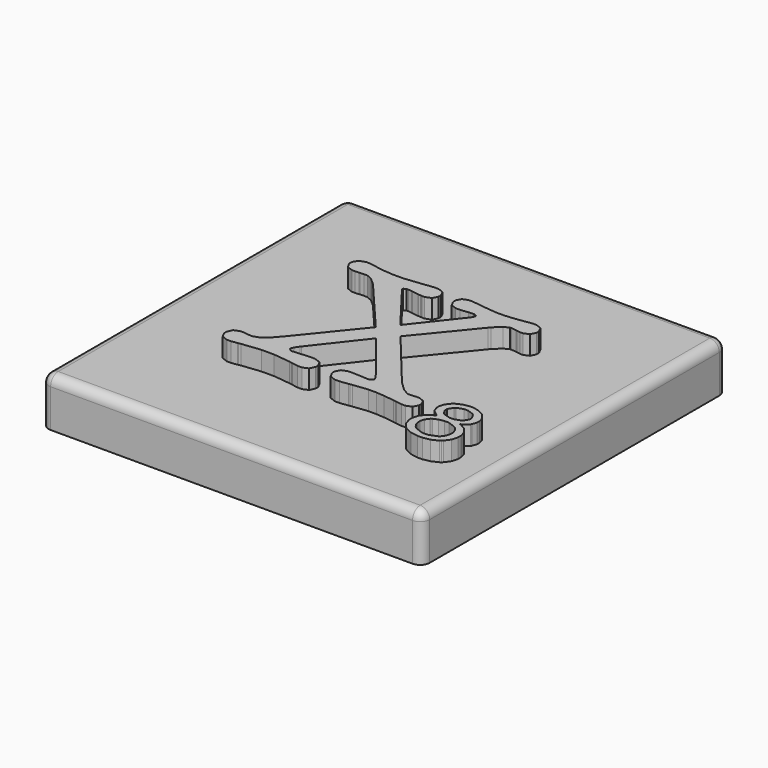
from build123d import *

# Parameters (mm, degrees)
F0_W     = 40
F0_H     = 40
F1_DEPTH = 5
F2_R     = 1
F5_DEPTH = 1
F6_DEPTH = 1
F7_DEPTH = 2


with BuildPart() as f1:
    # F0 (on Top) → F1 (new body)
    with BuildSketch(Plane.XY):
        Rectangle(F0_W, F0_H)
    extrude(amount=-F1_DEPTH)

    # F2
    f2_edges = [f1.edges().sort_by_distance(p)[0] for p in [
        (0, -20, 0),
        (20, 0, 0),
        (0, 20, 0),
        (-20, 0, 0),
        (-20, 20, -2.5),
        (20, 20, -2.5),
        (-20, -20, -2.5),
        (20, -20, -2.5),
    ]]
    fillet(f2_edges, radius=F2_R)

    # F3 (on Top) + F4 (on Top) → F5 (cut)
    with BuildSketch(Plane.XY):
        Polygon((-1.1913108, 0.4106672), (-5.873877, -5.3577998), (-6.0282328, -5.5465726), (-6.678676, -6.2921134), (-7.1651114, -6.7702938), (-7.2367648, -6.8254118), (-7.3098152, -6.8805298), (-8.0208628, -7.1561452), (-8.2813144, -7.1561452), (-8.3901788, -7.1561452), (-8.716772, -7.1230744), (-8.7719154, -7.1175626), (-8.8270334, -7.1106538), (-9.1398344, -7.077583), (-9.2611194, -7.077583), (-9.445752, -7.077583), (-9.9956112, -7.309104), (-10.239502, -7.8299818), (-10.239502, -8.0036416), (-10.239502, -8.1813908), (-9.962515, -8.7174578), (-9.3382846, -8.9558622), (-9.1288108, -8.9558622), (-8.9221056, -8.9558622), (-8.3006184, -8.8662764), (-8.2027776, -8.849741), (-7.960233, -8.8056466), (-6.0006738, -8.5851492), (-5.266182, -8.5851492), (-4.6722538, -8.5851492), (-2.8890722, -8.7835994), (-2.672715, -8.8235536), (-2.5541986, -8.8456008), (-1.8996406, -8.9558622), (-1.6405606, -8.9558622), (-1.4531594, -8.9558622), (-0.8881364, -8.7174578), (-0.6359906, -8.1813908), (-0.6359906, -8.0036416), (-0.6359906, -7.8299818), (-0.9267444, -7.309104), (-1.581277, -7.077583), (-1.7990058, -7.077583), (-1.9478498, -7.077583), (-2.394331, -7.0982586), (-2.4604726, -7.1037704), (-3.2542226, -7.1561452), (-3.86334, -7.2098916), (-3.9156894, -7.2098916), (-4.0094154, -7.2098916), (-4.286377, -6.9907658), (-4.286377, -6.9191124), (-4.286377, -6.8350638), (-4.167886, -6.5870074), (-3.8908736, -6.1722254), (-3.8109906, -6.071616), (0.0530606, -1.124458), (3.9942262, -6.071616), (4.0783002, -6.1763402), (4.371848, -6.6007742), (4.4972224, -6.8391786), (4.4972224, -6.9191124), (4.4972224, -6.985254), (4.1789096, -7.1837042), (4.07416, -7.1837042), (3.8895274, -7.1837042), (3.068193, -7.1299578), (2.9923994, -7.124446), (2.3943564, -7.1037704), (2.1697442, -7.1037704), (1.9657568, -7.1037704), (1.3553186, -7.3283826), (1.083818, -7.834122), (1.083818, -8.0036416), (1.083818, -8.1813908), (1.3676884, -8.7174578), (2.0084796, -8.9558622), (2.2220936, -8.9558622), (2.505964, -8.9558622), (3.3603692, -8.8456008), (3.4926524, -8.8235536), (3.7034724, -8.7877396), (5.2372514, -8.6113366), (5.8201306, -8.6113366), (6.0930028, -8.6113366), (6.9115686, -8.6705948), (8.0291178, -8.8097868), (8.2813144, -8.849741), (8.3915758, -8.8662764), (8.975852, -8.9558622), (9.207373, -8.9558622), (9.4003114, -8.9558622), (9.9804474, -8.7243412), (10.2395274, -8.203438), (10.2395274, -8.0298036), (10.2395274, -7.8658212), (9.9942396, -7.373874), (9.4430342, -7.1561452), (9.2597224, -7.1561452), (9.16051, -7.1561452), (8.8628474, -7.1781924), (8.83666, -7.1837042), (8.6781894, -7.1837042), (8.6561422, -7.187819), (8.5376258, -7.2098916), (8.4921344, -7.2098916), (8.256524, -7.2098916), (7.5537314, -6.8130166), (6.5918334, -5.886958), (6.3754762, -5.6223916), (1.4021562, 0.4106672), (6.058535, 6.0992258), (6.2128908, 6.2893702), (6.9115686, 6.952234), (7.4420984, 7.236079), (7.619873, 7.236079), (8.1131918, 7.1809864), (8.1752186, 7.1699374), (8.2358484, 7.1589392), (8.5913722, 7.1037958), (8.7305642, 7.1037958), (8.9138506, 7.1037958), (9.4650814, 7.3353168), (9.7103692, 7.85622), (9.7103692, 8.029829), (9.7103692, 8.2034634), (9.4374716, 8.724392), (8.8270334, 8.9558622), (8.624443, 8.9558622), (8.439785, 8.9558622), (7.8885796, 8.869045), (7.7783436, 8.8511634), (7.5302872, 8.8112092), (6.4609218, 8.6720172), (5.7223152, 8.612759), (5.4770274, 8.612759), (4.8913542, 8.612759), (3.1385002, 8.789162), (2.9358844, 8.823579), (2.8339542, 8.8415114), (2.182114, 8.9297002), (1.9313144, 8.9297002), (1.7466564, 8.9297002), (1.1954256, 8.7119714), (0.9515094, 8.2213958), (0.9515094, 8.0574134), (0.9515094, 7.883779), (1.2161012, 7.3628758), (1.8114264, 7.1313802), (2.0098512, 7.1313802), (2.2813518, 7.1313802), (3.0998922, 7.219569), (3.2280606, 7.236079), (3.2583628, 7.2416162), (3.5256978, 7.2636634), (3.6249356, 7.2636634), (3.7103812, 7.2636634), (3.9680642, 7.1051674), (3.9680642, 7.0514464), (3.9680642, 6.9439536), (3.7916612, 6.618732), (3.7572442, 6.5746122), (0.1315974, 1.9720052), (-3.5463988, 6.7868546), (-3.5725608, 6.822694), (-3.7048694, 7.025259), (-3.7048694, 7.1037958), (-3.7048694, 7.1506842), (-3.466465, 7.2898508), (-3.3865058, 7.2898508), (-3.2693864, 7.2898508), (-2.9138626, 7.2457564), (-2.8449778, 7.236079), (-2.7774392, 7.227824), (-2.1490432, 7.1410068), (-2.091182, 7.1313802), (-1.8527776, 7.1313802), (-1.8266156, 7.1272146), (-1.675003, 7.1037958), (-1.6143732, 7.1037958), (-1.415923, 7.1037958), (-0.8206232, 7.3353168), (-0.5560314, 7.85622), (-0.5560314, 8.029829), (-0.5560314, 8.1993486), (-0.8206232, 8.705088), (-1.415923, 8.9297002), (-1.6143732, 8.9297002), (-1.8238216, 8.9297002), (-2.4522176, 8.8649302), (-2.5404064, 8.8511634), (-2.8270454, 8.807069), (-4.8830738, 8.586597), (-5.663057, 8.586597), (-6.003417, 8.586597), (-7.0218046, 8.6747858), (-7.1444358, 8.6912958), (-7.4007472, 8.7353902), (-8.3281774, 8.8897206), (-8.69061, 8.9558622), (-8.810498, 8.9558622), (-9.0240866, 8.9558622), (-9.6648778, 8.732647), (-9.9487482, 8.2268822), (-9.9487482, 8.0574134), (-9.9487482, 7.8796642), (-9.6786446, 7.3435718), (-9.068181, 7.1037958), (-8.8642444, 7.1037958), (-8.7319358, 7.1037958), (-8.3336892, 7.1272146), (-8.2689192, 7.1313802), (-8.2055208, 7.135495), (-7.822438, 7.1575422), (-7.673594, 7.1575422), (-7.4793094, 7.1575422), (-6.8936362, 6.8929758), (-6.1825632, 6.2756034), (-6.0323476, 6.0992258), align=None)
    with BuildSketch(Plane.XY):
        Polygon((11.9091701338, -9.0316077608), (11.8678189338, -9.0633069608), (11.7562113338, -9.1487525608), (11.3675913338, -9.6696303608), (11.2022373338, -10.2649555608), (11.2022373338, -10.4633803608), (11.2022373338, -10.6728541608), (11.3772433338, -11.3039933608), (11.7879105338, -11.8648507608), (11.9064015338, -11.9585513608), (12.0235463338, -12.0522773608), (12.7277105338, -12.3802421608), (13.5187173338, -12.5208057608), (13.7833091338, -12.5208057608), (14.0368519338, -12.5208057608), (14.7989027338, -12.3774989608), (15.4851599338, -12.0439969608), (15.6023301338, -11.9489247608), (15.7180779338, -11.8538271608), (16.1232079338, -11.2915981608), (16.2968423338, -10.6700855608), (16.2968423338, -10.4633803608), (16.2968423338, -10.2635839608), (16.1301167338, -9.6655155608), (15.7414967338, -9.1473555608), (15.6312607338, -9.0633069608), (15.5871409338, -9.0316077608), (15.0400757338, -8.7449687608), (14.9739087338, -8.7201783608), (15.0593543338, -8.6705721608), (15.6505393338, -8.1978781608), (15.6836101338, -8.1537837608), (15.7153093338, -8.1083177608), (15.8779201338, -7.6287911608), (15.8779201338, -7.4537597608), (15.8779201338, -7.2870087608), (15.7235643338, -6.7881527608), (15.3652973338, -6.3209959608), (15.2632909338, -6.2397159608), (15.1599637338, -6.1570389608), (14.5784307338, -5.8703999608), (13.9596867338, -5.7491149608), (13.7543531338, -5.7491149608), (13.5476479338, -5.7491149608), (12.9289039338, -5.8703999608), (12.3459993338, -6.1570389608), (12.2440183338, -6.2397159608), (12.1406657338, -6.3209959608), (11.7837703338, -6.7881527608), (11.6308115338, -7.2870087608), (11.6308115338, -7.4537597608), (11.6308115338, -7.6163705608), (11.7892821338, -8.1083177608), (11.8209813338, -8.1537837608), (11.8526551338, -8.1978781608), (12.4466087338, -8.6705721608), (12.5347975338, -8.7201783608), (12.4645157338, -8.7449687608), align=None)
        Polygon((13.6096747338, -9.0825855608), (13.7929357338, -9.0825855608), (14.0754345338, -9.0825855608), (14.9243279338, -9.3954119608), (15.0014677338, -9.4588103608), (15.0772867338, -9.5208117608), (15.3446217338, -9.8956395608), (15.4589979338, -10.3131901608), (15.4589979338, -10.4537537608), (15.4589979338, -10.5929203608), (15.3404815338, -11.0146111608), (15.0662377338, -11.3935791608), (14.9877009338, -11.4583237608), (14.9091387338, -11.5217221608), (14.0616677338, -11.8441751608), (13.7543531338, -11.8441751608), (13.4649709338, -11.8441751608), (12.5995675338, -11.5217221608), (12.5210053338, -11.4583237608), (12.4424685338, -11.3935791608), (12.1668531338, -11.0146111608), (12.0497337338, -10.5929203608), (12.0497337338, -10.4537537608), (12.0497337338, -10.3104215608), (12.1641099338, -9.8832443608), (12.4341881338, -9.5097881608), (12.5113787338, -9.4491583608), (12.5871723338, -9.3871569608), (13.0612125338, -9.1735429608), align=None, mode=Mode.SUBTRACT)
        Polygon((13.5187173338, -6.4243485608), (13.7543531338, -6.4243485608), (13.9707103338, -6.4243485608), (14.6211535338, -6.6627783608), (14.6831549338, -6.7109875608), (14.7438101338, -6.7578505608), (15.0497277338, -7.2608213608), (15.0497277338, -7.4441077608), (15.0497277338, -7.5984381608), (14.7520651338, -8.0628263608), (14.6927815338, -8.1055491608), (14.6321771338, -8.1469003608), (13.9886173338, -8.3591427608), (13.7543531338, -8.3591427608), (13.5324841338, -8.3591427608), (12.8710427338, -8.1469003608), (12.8117845338, -8.1055491608), (12.7511547338, -8.0628263608), (12.4493519338, -7.6163705608), (12.4493519338, -7.4537597608), (12.4493519338, -7.2801253608), (12.7538979338, -6.7633369608), (12.8159247338, -6.7151277608), (12.8765545338, -6.6668931608), align=None, mode=Mode.SUBTRACT)
    extrude(amount=-F5_DEPTH, mode=Mode.SUBTRACT)


with BuildPart() as f6:
    # F3 (on Top) → F6 (new body)
    with BuildSketch(Plane.XY):
        Polygon((-1.1913108, 0.4106672), (-5.873877, -5.3577998), (-6.0282328, -5.5465726), (-6.678676, -6.2921134), (-7.1651114, -6.7702938), (-7.2367648, -6.8254118), (-7.3098152, -6.8805298), (-8.0208628, -7.1561452), (-8.2813144, -7.1561452), (-8.3901788, -7.1561452), (-8.716772, -7.1230744), (-8.7719154, -7.1175626), (-8.8270334, -7.1106538), (-9.1398344, -7.077583), (-9.2611194, -7.077583), (-9.445752, -7.077583), (-9.9956112, -7.309104), (-10.239502, -7.8299818), (-10.239502, -8.0036416), (-10.239502, -8.1813908), (-9.962515, -8.7174578), (-9.3382846, -8.9558622), (-9.1288108, -8.9558622), (-8.9221056, -8.9558622), (-8.3006184, -8.8662764), (-8.2027776, -8.849741), (-7.960233, -8.8056466), (-6.0006738, -8.5851492), (-5.266182, -8.5851492), (-4.6722538, -8.5851492), (-2.8890722, -8.7835994), (-2.672715, -8.8235536), (-2.5541986, -8.8456008), (-1.8996406, -8.9558622), (-1.6405606, -8.9558622), (-1.4531594, -8.9558622), (-0.8881364, -8.7174578), (-0.6359906, -8.1813908), (-0.6359906, -8.0036416), (-0.6359906, -7.8299818), (-0.9267444, -7.309104), (-1.581277, -7.077583), (-1.7990058, -7.077583), (-1.9478498, -7.077583), (-2.394331, -7.0982586), (-2.4604726, -7.1037704), (-3.2542226, -7.1561452), (-3.86334, -7.2098916), (-3.9156894, -7.2098916), (-4.0094154, -7.2098916), (-4.286377, -6.9907658), (-4.286377, -6.9191124), (-4.286377, -6.8350638), (-4.167886, -6.5870074), (-3.8908736, -6.1722254), (-3.8109906, -6.071616), (0.0530606, -1.124458), (3.9942262, -6.071616), (4.0783002, -6.1763402), (4.371848, -6.6007742), (4.4972224, -6.8391786), (4.4972224, -6.9191124), (4.4972224, -6.985254), (4.1789096, -7.1837042), (4.07416, -7.1837042), (3.8895274, -7.1837042), (3.068193, -7.1299578), (2.9923994, -7.124446), (2.3943564, -7.1037704), (2.1697442, -7.1037704), (1.9657568, -7.1037704), (1.3553186, -7.3283826), (1.083818, -7.834122), (1.083818, -8.0036416), (1.083818, -8.1813908), (1.3676884, -8.7174578), (2.0084796, -8.9558622), (2.2220936, -8.9558622), (2.505964, -8.9558622), (3.3603692, -8.8456008), (3.4926524, -8.8235536), (3.7034724, -8.7877396), (5.2372514, -8.6113366), (5.8201306, -8.6113366), (6.0930028, -8.6113366), (6.9115686, -8.6705948), (8.0291178, -8.8097868), (8.2813144, -8.849741), (8.3915758, -8.8662764), (8.975852, -8.9558622), (9.207373, -8.9558622), (9.4003114, -8.9558622), (9.9804474, -8.7243412), (10.2395274, -8.203438), (10.2395274, -8.0298036), (10.2395274, -7.8658212), (9.9942396, -7.373874), (9.4430342, -7.1561452), (9.2597224, -7.1561452), (9.16051, -7.1561452), (8.8628474, -7.1781924), (8.83666, -7.1837042), (8.6781894, -7.1837042), (8.6561422, -7.187819), (8.5376258, -7.2098916), (8.4921344, -7.2098916), (8.256524, -7.2098916), (7.5537314, -6.8130166), (6.5918334, -5.886958), (6.3754762, -5.6223916), (1.4021562, 0.4106672), (6.058535, 6.0992258), (6.2128908, 6.2893702), (6.9115686, 6.952234), (7.4420984, 7.236079), (7.619873, 7.236079), (8.1131918, 7.1809864), (8.1752186, 7.1699374), (8.2358484, 7.1589392), (8.5913722, 7.1037958), (8.7305642, 7.1037958), (8.9138506, 7.1037958), (9.4650814, 7.3353168), (9.7103692, 7.85622), (9.7103692, 8.029829), (9.7103692, 8.2034634), (9.4374716, 8.724392), (8.8270334, 8.9558622), (8.624443, 8.9558622), (8.439785, 8.9558622), (7.8885796, 8.869045), (7.7783436, 8.8511634), (7.5302872, 8.8112092), (6.4609218, 8.6720172), (5.7223152, 8.612759), (5.4770274, 8.612759), (4.8913542, 8.612759), (3.1385002, 8.789162), (2.9358844, 8.823579), (2.8339542, 8.8415114), (2.182114, 8.9297002), (1.9313144, 8.9297002), (1.7466564, 8.9297002), (1.1954256, 8.7119714), (0.9515094, 8.2213958), (0.9515094, 8.0574134), (0.9515094, 7.883779), (1.2161012, 7.3628758), (1.8114264, 7.1313802), (2.0098512, 7.1313802), (2.2813518, 7.1313802), (3.0998922, 7.219569), (3.2280606, 7.236079), (3.2583628, 7.2416162), (3.5256978, 7.2636634), (3.6249356, 7.2636634), (3.7103812, 7.2636634), (3.9680642, 7.1051674), (3.9680642, 7.0514464), (3.9680642, 6.9439536), (3.7916612, 6.618732), (3.7572442, 6.5746122), (0.1315974, 1.9720052), (-3.5463988, 6.7868546), (-3.5725608, 6.822694), (-3.7048694, 7.025259), (-3.7048694, 7.1037958), (-3.7048694, 7.1506842), (-3.466465, 7.2898508), (-3.3865058, 7.2898508), (-3.2693864, 7.2898508), (-2.9138626, 7.2457564), (-2.8449778, 7.236079), (-2.7774392, 7.227824), (-2.1490432, 7.1410068), (-2.091182, 7.1313802), (-1.8527776, 7.1313802), (-1.8266156, 7.1272146), (-1.675003, 7.1037958), (-1.6143732, 7.1037958), (-1.415923, 7.1037958), (-0.8206232, 7.3353168), (-0.5560314, 7.85622), (-0.5560314, 8.029829), (-0.5560314, 8.1993486), (-0.8206232, 8.705088), (-1.415923, 8.9297002), (-1.6143732, 8.9297002), (-1.8238216, 8.9297002), (-2.4522176, 8.8649302), (-2.5404064, 8.8511634), (-2.8270454, 8.807069), (-4.8830738, 8.586597), (-5.663057, 8.586597), (-6.003417, 8.586597), (-7.0218046, 8.6747858), (-7.1444358, 8.6912958), (-7.4007472, 8.7353902), (-8.3281774, 8.8897206), (-8.69061, 8.9558622), (-8.810498, 8.9558622), (-9.0240866, 8.9558622), (-9.6648778, 8.732647), (-9.9487482, 8.2268822), (-9.9487482, 8.0574134), (-9.9487482, 7.8796642), (-9.6786446, 7.3435718), (-9.068181, 7.1037958), (-8.8642444, 7.1037958), (-8.7319358, 7.1037958), (-8.3336892, 7.1272146), (-8.2689192, 7.1313802), (-8.2055208, 7.135495), (-7.822438, 7.1575422), (-7.673594, 7.1575422), (-7.4793094, 7.1575422), (-6.8936362, 6.8929758), (-6.1825632, 6.2756034), (-6.0323476, 6.0992258), align=None)
    extrude(amount=-F6_DEPTH)

    # F3 (on Top) → F7 (join)
    with BuildSketch(Plane.XY):
        Polygon((-1.1913108, 0.4106672), (-5.873877, -5.3577998), (-6.0282328, -5.5465726), (-6.678676, -6.2921134), (-7.1651114, -6.7702938), (-7.2367648, -6.8254118), (-7.3098152, -6.8805298), (-8.0208628, -7.1561452), (-8.2813144, -7.1561452), (-8.3901788, -7.1561452), (-8.716772, -7.1230744), (-8.7719154, -7.1175626), (-8.8270334, -7.1106538), (-9.1398344, -7.077583), (-9.2611194, -7.077583), (-9.445752, -7.077583), (-9.9956112, -7.309104), (-10.239502, -7.8299818), (-10.239502, -8.0036416), (-10.239502, -8.1813908), (-9.962515, -8.7174578), (-9.3382846, -8.9558622), (-9.1288108, -8.9558622), (-8.9221056, -8.9558622), (-8.3006184, -8.8662764), (-8.2027776, -8.849741), (-7.960233, -8.8056466), (-6.0006738, -8.5851492), (-5.266182, -8.5851492), (-4.6722538, -8.5851492), (-2.8890722, -8.7835994), (-2.672715, -8.8235536), (-2.5541986, -8.8456008), (-1.8996406, -8.9558622), (-1.6405606, -8.9558622), (-1.4531594, -8.9558622), (-0.8881364, -8.7174578), (-0.6359906, -8.1813908), (-0.6359906, -8.0036416), (-0.6359906, -7.8299818), (-0.9267444, -7.309104), (-1.581277, -7.077583), (-1.7990058, -7.077583), (-1.9478498, -7.077583), (-2.394331, -7.0982586), (-2.4604726, -7.1037704), (-3.2542226, -7.1561452), (-3.86334, -7.2098916), (-3.9156894, -7.2098916), (-4.0094154, -7.2098916), (-4.286377, -6.9907658), (-4.286377, -6.9191124), (-4.286377, -6.8350638), (-4.167886, -6.5870074), (-3.8908736, -6.1722254), (-3.8109906, -6.071616), (0.0530606, -1.124458), (3.9942262, -6.071616), (4.0783002, -6.1763402), (4.371848, -6.6007742), (4.4972224, -6.8391786), (4.4972224, -6.9191124), (4.4972224, -6.985254), (4.1789096, -7.1837042), (4.07416, -7.1837042), (3.8895274, -7.1837042), (3.068193, -7.1299578), (2.9923994, -7.124446), (2.3943564, -7.1037704), (2.1697442, -7.1037704), (1.9657568, -7.1037704), (1.3553186, -7.3283826), (1.083818, -7.834122), (1.083818, -8.0036416), (1.083818, -8.1813908), (1.3676884, -8.7174578), (2.0084796, -8.9558622), (2.2220936, -8.9558622), (2.505964, -8.9558622), (3.3603692, -8.8456008), (3.4926524, -8.8235536), (3.7034724, -8.7877396), (5.2372514, -8.6113366), (5.8201306, -8.6113366), (6.0930028, -8.6113366), (6.9115686, -8.6705948), (8.0291178, -8.8097868), (8.2813144, -8.849741), (8.3915758, -8.8662764), (8.975852, -8.9558622), (9.207373, -8.9558622), (9.4003114, -8.9558622), (9.9804474, -8.7243412), (10.2395274, -8.203438), (10.2395274, -8.0298036), (10.2395274, -7.8658212), (9.9942396, -7.373874), (9.4430342, -7.1561452), (9.2597224, -7.1561452), (9.16051, -7.1561452), (8.8628474, -7.1781924), (8.83666, -7.1837042), (8.6781894, -7.1837042), (8.6561422, -7.187819), (8.5376258, -7.2098916), (8.4921344, -7.2098916), (8.256524, -7.2098916), (7.5537314, -6.8130166), (6.5918334, -5.886958), (6.3754762, -5.6223916), (1.4021562, 0.4106672), (6.058535, 6.0992258), (6.2128908, 6.2893702), (6.9115686, 6.952234), (7.4420984, 7.236079), (7.619873, 7.236079), (8.1131918, 7.1809864), (8.1752186, 7.1699374), (8.2358484, 7.1589392), (8.5913722, 7.1037958), (8.7305642, 7.1037958), (8.9138506, 7.1037958), (9.4650814, 7.3353168), (9.7103692, 7.85622), (9.7103692, 8.029829), (9.7103692, 8.2034634), (9.4374716, 8.724392), (8.8270334, 8.9558622), (8.624443, 8.9558622), (8.439785, 8.9558622), (7.8885796, 8.869045), (7.7783436, 8.8511634), (7.5302872, 8.8112092), (6.4609218, 8.6720172), (5.7223152, 8.612759), (5.4770274, 8.612759), (4.8913542, 8.612759), (3.1385002, 8.789162), (2.9358844, 8.823579), (2.8339542, 8.8415114), (2.182114, 8.9297002), (1.9313144, 8.9297002), (1.7466564, 8.9297002), (1.1954256, 8.7119714), (0.9515094, 8.2213958), (0.9515094, 8.0574134), (0.9515094, 7.883779), (1.2161012, 7.3628758), (1.8114264, 7.1313802), (2.0098512, 7.1313802), (2.2813518, 7.1313802), (3.0998922, 7.219569), (3.2280606, 7.236079), (3.2583628, 7.2416162), (3.5256978, 7.2636634), (3.6249356, 7.2636634), (3.7103812, 7.2636634), (3.9680642, 7.1051674), (3.9680642, 7.0514464), (3.9680642, 6.9439536), (3.7916612, 6.618732), (3.7572442, 6.5746122), (0.1315974, 1.9720052), (-3.5463988, 6.7868546), (-3.5725608, 6.822694), (-3.7048694, 7.025259), (-3.7048694, 7.1037958), (-3.7048694, 7.1506842), (-3.466465, 7.2898508), (-3.3865058, 7.2898508), (-3.2693864, 7.2898508), (-2.9138626, 7.2457564), (-2.8449778, 7.236079), (-2.7774392, 7.227824), (-2.1490432, 7.1410068), (-2.091182, 7.1313802), (-1.8527776, 7.1313802), (-1.8266156, 7.1272146), (-1.675003, 7.1037958), (-1.6143732, 7.1037958), (-1.415923, 7.1037958), (-0.8206232, 7.3353168), (-0.5560314, 7.85622), (-0.5560314, 8.029829), (-0.5560314, 8.1993486), (-0.8206232, 8.705088), (-1.415923, 8.9297002), (-1.6143732, 8.9297002), (-1.8238216, 8.9297002), (-2.4522176, 8.8649302), (-2.5404064, 8.8511634), (-2.8270454, 8.807069), (-4.8830738, 8.586597), (-5.663057, 8.586597), (-6.003417, 8.586597), (-7.0218046, 8.6747858), (-7.1444358, 8.6912958), (-7.4007472, 8.7353902), (-8.3281774, 8.8897206), (-8.69061, 8.9558622), (-8.810498, 8.9558622), (-9.0240866, 8.9558622), (-9.6648778, 8.732647), (-9.9487482, 8.2268822), (-9.9487482, 8.0574134), (-9.9487482, 7.8796642), (-9.6786446, 7.3435718), (-9.068181, 7.1037958), (-8.8642444, 7.1037958), (-8.7319358, 7.1037958), (-8.3336892, 7.1272146), (-8.2689192, 7.1313802), (-8.2055208, 7.135495), (-7.822438, 7.1575422), (-7.673594, 7.1575422), (-7.4793094, 7.1575422), (-6.8936362, 6.8929758), (-6.1825632, 6.2756034), (-6.0323476, 6.0992258), align=None)
    extrude(amount=F7_DEPTH)


with BuildPart() as f6b:
    # F4 (on Top) → F6, piece 2 (new body)
    with BuildSketch(Plane.XY):
        Polygon((11.9091701338, -9.0316077608), (11.8678189338, -9.0633069608), (11.7562113338, -9.1487525608), (11.3675913338, -9.6696303608), (11.2022373338, -10.2649555608), (11.2022373338, -10.4633803608), (11.2022373338, -10.6728541608), (11.3772433338, -11.3039933608), (11.7879105338, -11.8648507608), (11.9064015338, -11.9585513608), (12.0235463338, -12.0522773608), (12.7277105338, -12.3802421608), (13.5187173338, -12.5208057608), (13.7833091338, -12.5208057608), (14.0368519338, -12.5208057608), (14.7989027338, -12.3774989608), (15.4851599338, -12.0439969608), (15.6023301338, -11.9489247608), (15.7180779338, -11.8538271608), (16.1232079338, -11.2915981608), (16.2968423338, -10.6700855608), (16.2968423338, -10.4633803608), (16.2968423338, -10.2635839608), (16.1301167338, -9.6655155608), (15.7414967338, -9.1473555608), (15.6312607338, -9.0633069608), (15.5871409338, -9.0316077608), (15.0400757338, -8.7449687608), (14.9739087338, -8.7201783608), (15.0593543338, -8.6705721608), (15.6505393338, -8.1978781608), (15.6836101338, -8.1537837608), (15.7153093338, -8.1083177608), (15.8779201338, -7.6287911608), (15.8779201338, -7.4537597608), (15.8779201338, -7.2870087608), (15.7235643338, -6.7881527608), (15.3652973338, -6.3209959608), (15.2632909338, -6.2397159608), (15.1599637338, -6.1570389608), (14.5784307338, -5.8703999608), (13.9596867338, -5.7491149608), (13.7543531338, -5.7491149608), (13.5476479338, -5.7491149608), (12.9289039338, -5.8703999608), (12.3459993338, -6.1570389608), (12.2440183338, -6.2397159608), (12.1406657338, -6.3209959608), (11.7837703338, -6.7881527608), (11.6308115338, -7.2870087608), (11.6308115338, -7.4537597608), (11.6308115338, -7.6163705608), (11.7892821338, -8.1083177608), (11.8209813338, -8.1537837608), (11.8526551338, -8.1978781608), (12.4466087338, -8.6705721608), (12.5347975338, -8.7201783608), (12.4645157338, -8.7449687608), align=None)
        Polygon((13.6096747338, -9.0825855608), (13.7929357338, -9.0825855608), (14.0754345338, -9.0825855608), (14.9243279338, -9.3954119608), (15.0014677338, -9.4588103608), (15.0772867338, -9.5208117608), (15.3446217338, -9.8956395608), (15.4589979338, -10.3131901608), (15.4589979338, -10.4537537608), (15.4589979338, -10.5929203608), (15.3404815338, -11.0146111608), (15.0662377338, -11.3935791608), (14.9877009338, -11.4583237608), (14.9091387338, -11.5217221608), (14.0616677338, -11.8441751608), (13.7543531338, -11.8441751608), (13.4649709338, -11.8441751608), (12.5995675338, -11.5217221608), (12.5210053338, -11.4583237608), (12.4424685338, -11.3935791608), (12.1668531338, -11.0146111608), (12.0497337338, -10.5929203608), (12.0497337338, -10.4537537608), (12.0497337338, -10.3104215608), (12.1641099338, -9.8832443608), (12.4341881338, -9.5097881608), (12.5113787338, -9.4491583608), (12.5871723338, -9.3871569608), (13.0612125338, -9.1735429608), align=None, mode=Mode.SUBTRACT)
        Polygon((13.5187173338, -6.4243485608), (13.7543531338, -6.4243485608), (13.9707103338, -6.4243485608), (14.6211535338, -6.6627783608), (14.6831549338, -6.7109875608), (14.7438101338, -6.7578505608), (15.0497277338, -7.2608213608), (15.0497277338, -7.4441077608), (15.0497277338, -7.5984381608), (14.7520651338, -8.0628263608), (14.6927815338, -8.1055491608), (14.6321771338, -8.1469003608), (13.9886173338, -8.3591427608), (13.7543531338, -8.3591427608), (13.5324841338, -8.3591427608), (12.8710427338, -8.1469003608), (12.8117845338, -8.1055491608), (12.7511547338, -8.0628263608), (12.4493519338, -7.6163705608), (12.4493519338, -7.4537597608), (12.4493519338, -7.2801253608), (12.7538979338, -6.7633369608), (12.8159247338, -6.7151277608), (12.8765545338, -6.6668931608), align=None, mode=Mode.SUBTRACT)
    extrude(amount=-F6_DEPTH)

    # F4 (on Top) → F7, piece 2 (join)
    with BuildSketch(Plane.XY):
        Polygon((11.9091701338, -9.0316077608), (11.8678189338, -9.0633069608), (11.7562113338, -9.1487525608), (11.3675913338, -9.6696303608), (11.2022373338, -10.2649555608), (11.2022373338, -10.4633803608), (11.2022373338, -10.6728541608), (11.3772433338, -11.3039933608), (11.7879105338, -11.8648507608), (11.9064015338, -11.9585513608), (12.0235463338, -12.0522773608), (12.7277105338, -12.3802421608), (13.5187173338, -12.5208057608), (13.7833091338, -12.5208057608), (14.0368519338, -12.5208057608), (14.7989027338, -12.3774989608), (15.4851599338, -12.0439969608), (15.6023301338, -11.9489247608), (15.7180779338, -11.8538271608), (16.1232079338, -11.2915981608), (16.2968423338, -10.6700855608), (16.2968423338, -10.4633803608), (16.2968423338, -10.2635839608), (16.1301167338, -9.6655155608), (15.7414967338, -9.1473555608), (15.6312607338, -9.0633069608), (15.5871409338, -9.0316077608), (15.0400757338, -8.7449687608), (14.9739087338, -8.7201783608), (15.0593543338, -8.6705721608), (15.6505393338, -8.1978781608), (15.6836101338, -8.1537837608), (15.7153093338, -8.1083177608), (15.8779201338, -7.6287911608), (15.8779201338, -7.4537597608), (15.8779201338, -7.2870087608), (15.7235643338, -6.7881527608), (15.3652973338, -6.3209959608), (15.2632909338, -6.2397159608), (15.1599637338, -6.1570389608), (14.5784307338, -5.8703999608), (13.9596867338, -5.7491149608), (13.7543531338, -5.7491149608), (13.5476479338, -5.7491149608), (12.9289039338, -5.8703999608), (12.3459993338, -6.1570389608), (12.2440183338, -6.2397159608), (12.1406657338, -6.3209959608), (11.7837703338, -6.7881527608), (11.6308115338, -7.2870087608), (11.6308115338, -7.4537597608), (11.6308115338, -7.6163705608), (11.7892821338, -8.1083177608), (11.8209813338, -8.1537837608), (11.8526551338, -8.1978781608), (12.4466087338, -8.6705721608), (12.5347975338, -8.7201783608), (12.4645157338, -8.7449687608), align=None)
        Polygon((13.6096747338, -9.0825855608), (13.7929357338, -9.0825855608), (14.0754345338, -9.0825855608), (14.9243279338, -9.3954119608), (15.0014677338, -9.4588103608), (15.0772867338, -9.5208117608), (15.3446217338, -9.8956395608), (15.4589979338, -10.3131901608), (15.4589979338, -10.4537537608), (15.4589979338, -10.5929203608), (15.3404815338, -11.0146111608), (15.0662377338, -11.3935791608), (14.9877009338, -11.4583237608), (14.9091387338, -11.5217221608), (14.0616677338, -11.8441751608), (13.7543531338, -11.8441751608), (13.4649709338, -11.8441751608), (12.5995675338, -11.5217221608), (12.5210053338, -11.4583237608), (12.4424685338, -11.3935791608), (12.1668531338, -11.0146111608), (12.0497337338, -10.5929203608), (12.0497337338, -10.4537537608), (12.0497337338, -10.3104215608), (12.1641099338, -9.8832443608), (12.4341881338, -9.5097881608), (12.5113787338, -9.4491583608), (12.5871723338, -9.3871569608), (13.0612125338, -9.1735429608), align=None, mode=Mode.SUBTRACT)
        Polygon((13.5187173338, -6.4243485608), (13.7543531338, -6.4243485608), (13.9707103338, -6.4243485608), (14.6211535338, -6.6627783608), (14.6831549338, -6.7109875608), (14.7438101338, -6.7578505608), (15.0497277338, -7.2608213608), (15.0497277338, -7.4441077608), (15.0497277338, -7.5984381608), (14.7520651338, -8.0628263608), (14.6927815338, -8.1055491608), (14.6321771338, -8.1469003608), (13.9886173338, -8.3591427608), (13.7543531338, -8.3591427608), (13.5324841338, -8.3591427608), (12.8710427338, -8.1469003608), (12.8117845338, -8.1055491608), (12.7511547338, -8.0628263608), (12.4493519338, -7.6163705608), (12.4493519338, -7.4537597608), (12.4493519338, -7.2801253608), (12.7538979338, -6.7633369608), (12.8159247338, -6.7151277608), (12.8765545338, -6.6668931608), align=None, mode=Mode.SUBTRACT)
    extrude(amount=F7_DEPTH)


solid = Compound([f1.part, f6.part, f6b.part])
